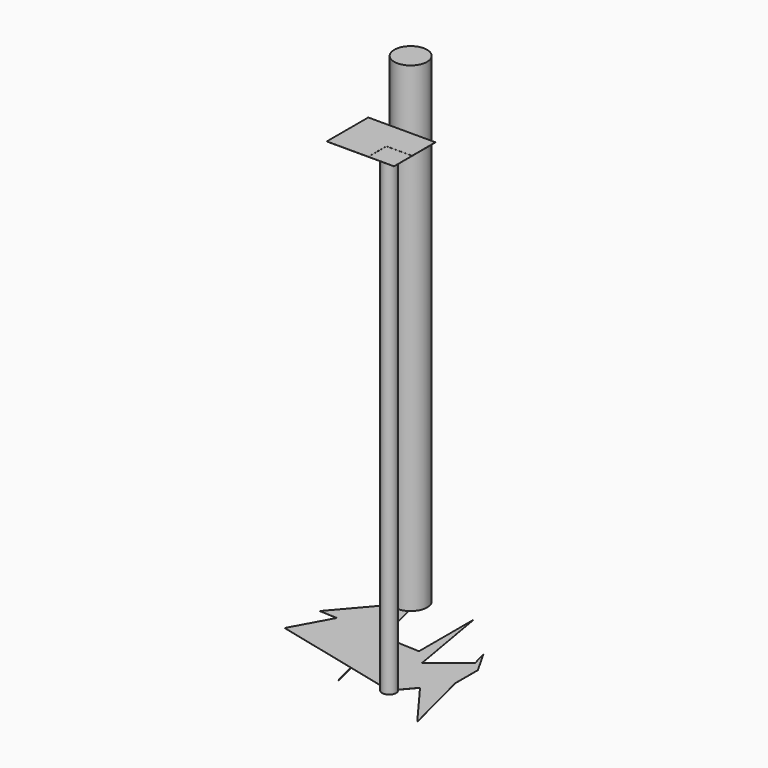
from build123d import *

# Parameters (mm, degrees)
F0_R      = 2235.2
F1_DEPTH  = 152400
F2_W      = 16314.079284668
F2_H      = 16430.6888580322
F3_DEPTH  = 25.4
F4_W      = 13162.3058319092
F4_H      = 7196.5775489807
F5_DEPTH  = 25.4
F6_R      = 5206.746363133
F7_DEPTH  = 152400
F8_W      = 130.4168701172
F8_H      = 3464.111328125
F9_DEPTH  = 25.4
F10_DEPTH = 25.4


with BuildPart() as f1:
    # F0 (on Top) → F1 (new body)
    with BuildSketch(Plane.XY):
        Circle(F0_R)
    extrude(amount=F1_DEPTH)

    # F2 (on face) → F3 (join)
    with BuildSketch(Plane.XY.offset(152400)):
        with Locations((-2.9983520508, -39.6871566772)):
            Rectangle(F2_W, F2_H)
    extrude(amount=F3_DEPTH)

    # F4 (on face) → F5 (join)
    with BuildSketch(Plane.XY.offset(152425.4)):
        with Locations((-6581.1529159546, -4679.9094676971)):
            Rectangle(F4_W, F4_H)
        Polygon((-13162.3058319092, -1081.6206932068), (0, -1081.6206932068), (8154.0412902832, -1081.6206932068), (8154.0412902832, 8175.6572723389), (-13162.3058319092, 8175.6572723389), align=None)
    extrude(amount=F5_DEPTH)


with BuildPart() as f7:
    # F6 (on face) → F7 (new body, through all)
    with BuildSketch(Plane(origin=(0, 0, 152400), x_dir=(1, 0, 0), z_dir=(0, 0, -1))):
        with Locations((-25685.0719451904, -40658.6380004883)):
            Circle(F6_R)
    extrude(amount=F7_DEPTH)


with BuildPart() as f9:
    # F8 (on face) → F9 (new body)
    with BuildSketch(Plane(origin=(0, 0, 0), x_dir=(1, 0, 0), z_dir=(0, 0, -1))):
        with Locations((-24038.5856628418, -39383.0947875977)):
            Rectangle(F8_W, F8_H)
        Polygon((-34421.4778333763, -22294.6625748956), (-24103.7940979004, -41115.1504516602), (-24103.7940979004, -37651.0391235352), (-23973.3772277832, -37651.0391235352), (-19811.9348288427, -21624.8610825982), align=None)
        Polygon((-40052.1812438965, -22552.8125762939), (-24103.7940979004, -41115.1504516602), (-34421.4778333763, -22294.6625748956), align=None)
        Polygon((-23973.3772277832, -37651.0391235352), (-23973.3772277832, -41115.1504516602), (-19260.1197917863, -21599.5621026658), (-19811.9348288427, -21624.8610825982), align=None)
        Polygon((-41149.227142334, -10022.5744247436), (-34421.4778333763, -22294.6625748956), (-19811.9348288427, -21624.8610825982), (-16222.995959886, -7803.457881972), align=None)
        Polygon((-15921.7109515854, -7776.6352732464), (-19260.1197917863, -21599.5621026658), (-7381.2336921692, -21054.95262146), (-2301.1527002977, -6564.0329381408), align=None)
        Polygon((-19811.9348288427, -21624.8610825982), (-19260.1197917863, -21599.5621026658), (-15921.7109515854, -7776.6352732464), (-16222.995959886, -7803.457881972), align=None)
        Polygon((-15155.2118404192, -3691.3023437344), (-41149.227142334, -10022.5744247437), (-16222.995959886, -7803.457881972), align=None)
        Polygon((-2301.1527002977, -6564.0329381408), (-7381.2336921692, -21054.95262146), (-7381.2336921692, -42754.9171447754), (-2874.0796962277, -16647.7643717013), (-1114.9874071605, -6458.4317742426), align=None)
        Polygon((-16222.995959886, -7803.457881972), (-15921.7109515854, -7776.6352732464), (-14921.2920315378, -3634.3273078285), (-15155.2118404192, -3691.3023437344), align=None)
        Polygon((-14921.2920315378, -3634.3273078285), (-15921.7109515854, -7776.6352732464), (-2301.1527002977, -6564.0329381408), (0, 0), align=None)
        Polygon((-12005.9661865234, 8436.7933273315), (-15155.2118404192, -3691.3023437344), (-14921.2920315378, -3634.3273078285), align=None)
        Polygon((0, 0), (-2301.1527002977, -6564.0329381408), (-1114.9874071605, -6458.4317742426), align=None)
        Polygon((5075.7439402199, -5907.2873094308), (-2874.0796962277, -16647.7643717013), (10348.1292724609, -12262.6476287842), (10348.1292724609, -13251.1214584158), (15950.0694274902, 8784.2893600464), align=None)
        Polygon((-1114.9874071605, -6458.4317742426), (-2874.0796962277, -16647.7643717013), (5075.7439402199, -5907.2873094308), align=None)
        Polygon((10348.1292724609, -12262.6476287842), (-2874.0796962277, -16647.7643717013), (7441.0890589714, -24686.057140926), (10348.1292724609, -13251.1214584158), align=None)
        Polygon((5075.7439402199, -5907.2873094308), (0, 0), (-1114.9874071605, -6458.4317742426), align=None)
        Polygon((10348.1292724609, -13251.1214584158), (7441.0890589715, -24686.057140926), (6189.8880004883, -29607.6965332031), (10348.1292724609, -22246.000289917), (10348.1292724609, -14536.7050170898), align=None)
    extrude(amount=F9_DEPTH)


with BuildPart() as f10:
    # F0 (on Top) → F10 (new body)
    with BuildSketch(Plane.XY):
        Circle(F0_R)
    extrude(amount=F10_DEPTH)


solid = Compound([f1.part, f7.part, f9.part, f10.part])
